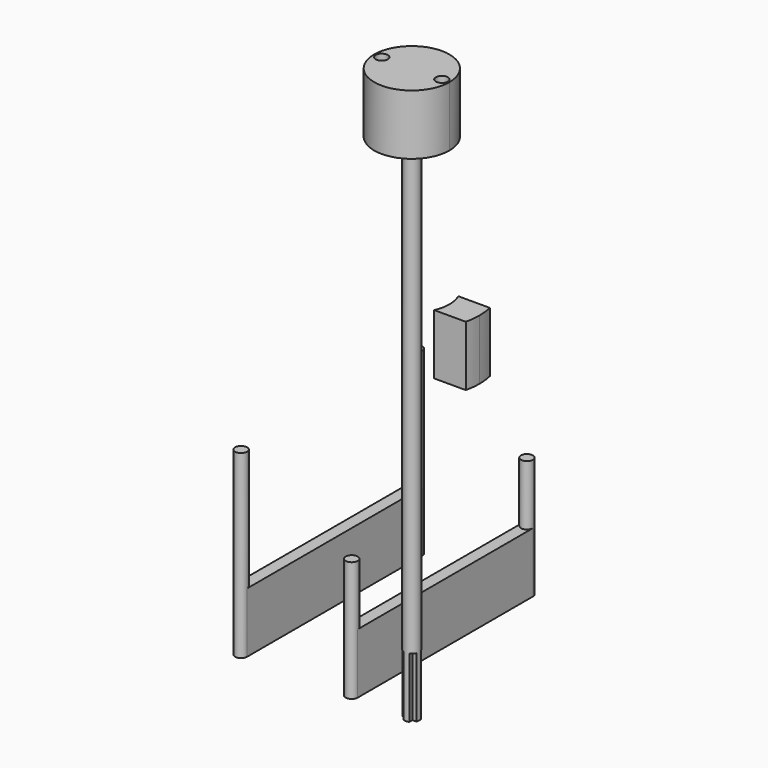
from build123d import *

# Parameters (mm, degrees)
F0_R      = 0.635
F1_DEPTH  = 48.26
F3_DEPTH  = 5.08
F5_DEPTH  = 5.08
F6_R      = 0.508
F7_DEPTH  = 5.08
F8_R      = 0.508
F9_DEPTH  = 10.16
F12_DEPTH = 5.08
F14_DEPTH = 5.08


with BuildPart() as f1:
    # F0 (on Top) → F1 (new body)
    with BuildSketch(Plane.XY):
        Circle(F0_R)
    extrude(amount=F1_DEPTH)

    # F2 (on face) → F3 (join)
    with BuildSketch(Plane.XY.offset(48.26)):
        with BuildLine():
            Line((3.048, 0), (3.175, 0))
            ThreePointArc((3.175, 0), (2.2450640303, 2.2450640303), (0, 3.175))
            Line((0, 3.175), (0, 0))
            Line((0, 0), (2.032, 0))
            ThreePointArc((2.032, 0), (2.54, 0.508), (3.048, 0))
        make_face()
        with BuildLine():
            ThreePointArc((-3.175, 0), (0, -3.175), (3.175, 0))
            Line((3.175, 0), (3.048, 0))
            ThreePointArc((3.048, 0), (2.54, -0.508), (2.032, 0))
            Line((2.032, 0), (0, 0))
            Line((0, 0), (-2.032, 0))
            ThreePointArc((-2.032, 0), (-2.54, -0.508), (-3.048, 0))
            Line((-3.048, 0), (-3.175, 0))
        make_face()
        with BuildLine():
            Line((0, 0), (0, 3.175))
            ThreePointArc((0, 3.175), (-2.2450640303, 2.2450640303), (-3.175, 0))
            Line((-3.175, 0), (-3.048, 0))
            ThreePointArc((-3.048, 0), (-2.54, 0.508), (-2.032, 0))
            Line((-2.032, 0), (0, 0))
        make_face()
    extrude(amount=-F3_DEPTH)

    # F13 (on face) → F14 (cut)
    with BuildSketch(Plane(origin=(0, 0, 0), x_dir=(1, 0, 0), z_dir=(0, 0, -1))):
        with BuildLine():
            Line((0.254, 0.254), (0.5819871133, 0.254))
            ThreePointArc((0.5819871133, 0.254), (0.4490128061, 0.4490128061), (0.254, 0.5819871133))
            Line((0.254, 0.5819871133), (0.254, 0.254))
        make_face()
        with BuildLine():
            ThreePointArc((0.254, -0.5819871133), (0.4490128061, -0.4490128061), (0.5819871133, -0.254))
            Line((0.5819871133, -0.254), (0.254, -0.254))
            Line((0.254, -0.254), (0.254, -0.5819871133))
        make_face()
        with BuildLine():
            ThreePointArc((-0.254, 0.5819871133), (0, 0.635), (0.254, 0.5819871133))
            Line((0.254, 0.5819871133), (0.254, 4.8890965991))
            Line((0.254, 4.8890965991), (-0.254, 4.8890965991))
            Line((-0.254, 4.8890965991), (-0.254, 0.5819871133))
        make_face()
        with BuildLine():
            Line((0.254, -4.8890965991), (0.254, -0.5819871133))
            ThreePointArc((0.254, -0.5819871133), (0, -0.635), (-0.254, -0.5819871133))
            Line((-0.254, -0.5819871133), (-0.254, -4.8890965991))
            Line((-0.254, -4.8890965991), (0.254, -4.8890965991))
        make_face()
        with BuildLine():
            Line((-0.254, 0.254), (-0.254, 0.5819871133))
            ThreePointArc((-0.254, 0.5819871133), (-0.4490128061, 0.4490128061), (-0.5819871133, 0.254))
            Line((-0.5819871133, 0.254), (-0.254, 0.254))
        make_face()
        with BuildLine():
            ThreePointArc((-0.5819871133, -0.254), (-0.4490128061, -0.4490128061), (-0.254, -0.5819871133))
            Line((-0.254, -0.5819871133), (-0.254, -0.254))
            Line((-0.254, -0.254), (-0.5819871133, -0.254))
        make_face()
    extrude(amount=-F14_DEPTH, mode=Mode.SUBTRACT)


with BuildPart() as f5:
    # F4 (on Top) → F5 (new body)
    with BuildSketch(Plane.XY):
        with BuildLine():
            ThreePointArc((-5.5828010944, 0), (-5.0748010944, -0.508), (-4.5668010944, 0))
            Line((-4.5668010944, 0), (-5.5828010944, 0))
        make_face()
        with BuildLine():
            ThreePointArc((-5.5828010944, 0), (-5.0748010944, 0.508), (-4.5668010944, 0))
            Line((-4.5668010944, 0), (-4.5668010944, 18.4914791188))
            ThreePointArc((-4.5668010944, 18.4914791188), (-5.0748010944, 17.9834791188), (-5.5828010944, 18.4914791188))
            Line((-5.5828010944, 18.4914791188), (-5.5828010944, 0))
        make_face()
        with BuildLine():
            Line((-5.5828010944, 0), (-4.5668010944, 0))
            ThreePointArc((-4.5668010944, 0), (-5.0748010944, 0.508), (-5.5828010944, 0))
        make_face()
        with BuildLine():
            ThreePointArc((-5.5828010944, 18.4914791188), (-5.0748010944, 17.9834791188), (-4.5668010944, 18.4914791188))
            Line((-4.5668010944, 18.4914791188), (-5.5828010944, 18.4914791188))
        make_face()
        with BuildLine():
            Line((-5.5828010944, 18.4914791188), (-4.5668010944, 18.4914791188))
            ThreePointArc((-4.5668010944, 18.4914791188), (-5.0748010944, 18.9994791188), (-5.5828010944, 18.4914791188))
        make_face()
    extrude(amount=F5_DEPTH)

    # F6 (on face) → F7 (join)
    with BuildSketch(Plane.XY.offset(5.08)):
        with Locations((-5.0748010944, 18.4914791188)):
            Circle(F6_R)
        with Locations((-5.0748010944, 0)):
            Circle(F6_R)
    extrude(amount=F7_DEPTH)


with BuildPart() as f5b:
    # F4 (on Top) → F5, piece 2 (new body)
    with BuildSketch(Plane.XY):
        with BuildLine():
            ThreePointArc((-14.9213979021, 0), (-14.4133979021, -0.508), (-13.9053979021, 0))
            Line((-13.9053979021, 0), (-14.4133979021, 0))
            Line((-14.4133979021, 0), (-14.9213979021, 0))
        make_face()
        with BuildLine():
            Line((-14.4133979021, 0), (-13.9053979021, 0))
            ThreePointArc((-13.9053979021, 0), (-14.4133979021, 0.508), (-14.9213979021, 0))
            Line((-14.9213979021, 0), (-14.4133979021, 0))
        make_face()
        with BuildLine():
            ThreePointArc((-14.9213979021, 0), (-14.4133979021, 0.508), (-13.9053979021, 0))
            Line((-13.9053979021, 0), (-13.9053979021, 18.4914791188))
            ThreePointArc((-13.9053979021, 18.4914791188), (-14.4133979021, 17.9834791188), (-14.9213979021, 18.4914791188))
            Line((-14.9213979021, 18.4914791188), (-14.9213979021, 0))
        make_face()
        with BuildLine():
            ThreePointArc((-14.9213979021, 18.4914791188), (-14.4133979021, 17.9834791188), (-13.9053979021, 18.4914791188))
            Line((-13.9053979021, 18.4914791188), (-14.9213979021, 18.4914791188))
        make_face()
        with BuildLine():
            Line((-14.9213979021, 18.4914791188), (-13.9053979021, 18.4914791188))
            ThreePointArc((-13.9053979021, 18.4914791188), (-14.4133979021, 18.9994791188), (-14.9213979021, 18.4914791188))
        make_face()
    extrude(amount=F5_DEPTH)

    # F8 (on face) → F9 (join)
    with BuildSketch(Plane.XY.offset(5.08)):
        with Locations((-14.4133979021, 18.4914791188)):
            Circle(F8_R)
        with Locations((-14.4133979021, 0)):
            Circle(F8_R)
    extrude(amount=F9_DEPTH)


with BuildPart() as f12:
    # F11 (on offset) → F12 (new body)
    with BuildSketch(Plane.XY.offset(31.75)):
        with BuildLine():
            ThreePointArc((2.9099355663, 1.27), (3.1080275436, 0.6486831187), (3.175, 0))
            ThreePointArc((3.175, 0), (3.1080275436, -0.6486831187), (2.9099355663, -1.27))
            Line((2.9099355663, -1.27), (5.572102386, -1.27))
            Line((5.572102386, -1.27), (5.572102386, 1.27))
            Line((5.572102386, 1.27), (2.9099355663, 1.27))
        make_face()
        with BuildLine():
            ThreePointArc((5.715, 0), (5.6791632366, 0.639006989), (5.572102386, 1.27))
            Line((5.572102386, 1.27), (5.572102386, -1.27))
            ThreePointArc((5.572102386, -1.27), (5.6791632366, -0.639006989), (5.715, 0))
        make_face()
    extrude(amount=-F12_DEPTH)


solid = Compound([f1.part, f5.part, f5b.part, f12.part])
